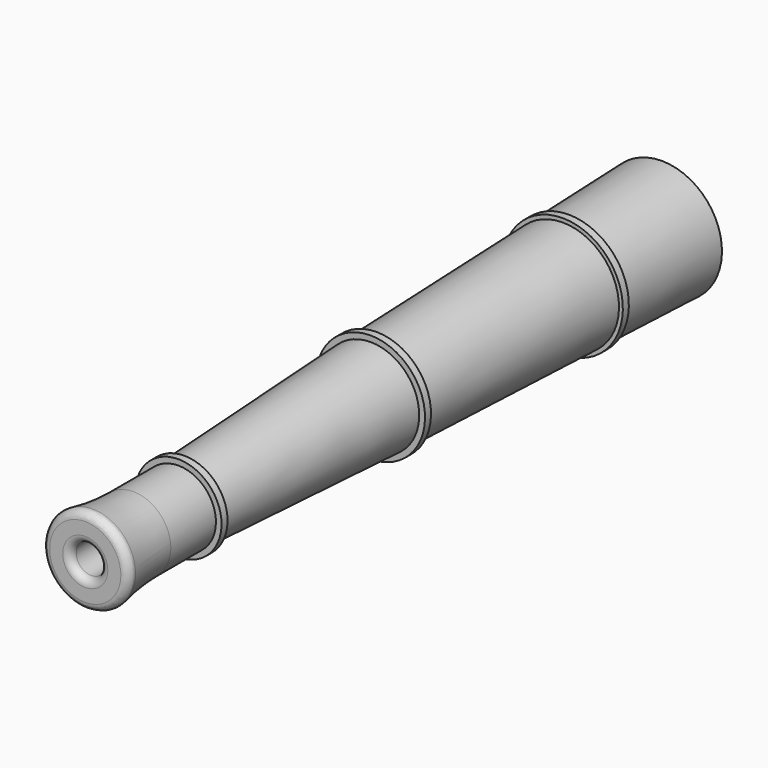
from build123d import *

# Parameters (mm, degrees)
F2_R = 0.79375


with BuildPart() as f1:
    # F0 (on Right) → F1 (revolve)
    with BuildSketch(Plane.YZ):
        with BuildLine():
            Line((0, 1.5875), (12.303125, 1.5875))
            Line((12.303125, 1.5875), (12.303125, 3.96875))
            Line((12.303125, 3.96875), (6.35, 3.96875))
            ThreePointArc((6.35, 3.96875), (3.1502914561, 4.1679566492), (0, 4.7625))
            Line((0, 4.7625), (0, 1.5875))
        make_face()
        Polygon((12.303125, 1.5875), (13.096875, 1.5875), (13.096875, 3.9873535156), (12.7, 3.96875), (12.303125, 3.96875), align=None)
        Polygon((12.7, 3.96875), (13.096875, 3.9873535156), (13.096875, 4.5640625), (12.303125, 4.5640625), (12.303125, 3.96875), align=None)
        Polygon((13.096875, 1.5875), (37.703125, 1.5875), (37.703125, 5.1407714844), (13.096875, 3.9873535156), align=None)
        Polygon((37.703125, 1.5875), (38.496875, 1.5875), (38.496875, 5.1717773437), (38.1, 5.159375), (37.703125, 5.1407714844), align=None)
        Polygon((38.1, 5.159375), (38.496875, 5.1717773437), (38.496875, 5.7546875), (37.703125, 5.7546875), (37.703125, 5.1407714844), align=None)
        Polygon((38.496875, 1.5875), (63.103125, 1.5875), (63.103125, 5.9407226563), (38.496875, 5.1717773437), align=None)
        Polygon((63.896875, 1.5875), (76.2, 1.5875), (76.2, 6.35), (63.896875, 5.9655273437), align=None)
        Polygon((63.103125, 1.5875), (63.896875, 1.5875), (63.896875, 5.9655273437), (63.5, 5.953125), (63.103125, 5.9407226563), align=None)
        Polygon((63.5, 5.953125), (63.896875, 5.9655273437), (63.896875, 6.35), (63.103125, 6.35), (63.103125, 5.9407226563), align=None)
    revolve(axis=Axis((0, 38.1, 0), (0, 1, 0)))

    # F2
    f2_edges = [f1.edges().sort_by_distance(p)[0] for p in [
        (0, 0, -4.7625),
        (0, 0, -1.5875),
    ]]
    fillet(f2_edges, radius=F2_R)


solid = f1.part
